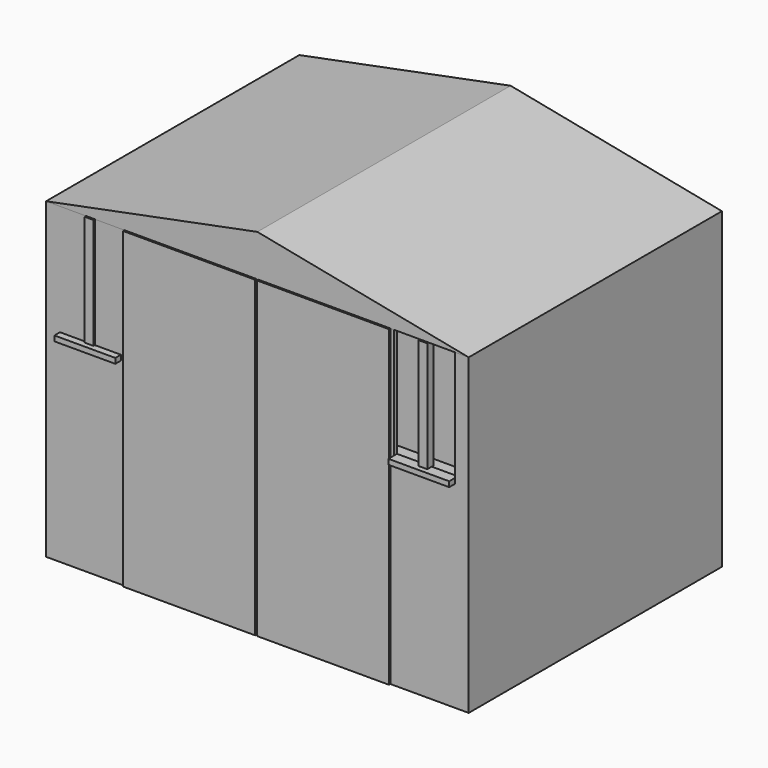
from build123d import *

# Parameters (mm, degrees)
F0_W          = 243
F0_H          = 182
F0_W_2        = 238.6
F0_H_2        = 177.6
F1_DEPTH      = 180
F2_DEPTH      = 2.2
F3_W          = 76
F3_H          = 180
F3_W_2        = 5
F3_H_2        = 63.7124854326
F4_DEPTH      = 1
F4_DEPTH_BACK = 3.3
F3_W_3        = 15
F5_DEPTH      = 25
F6_DEPTH      = 8
F7_DEPTH      = 4
F9_DEPTH      = 182


# Not quite as in the source:
# - a feature names something its author has since deleted; it is built from what else it names


with BuildPart() as f1:
    # F0 (on Top) → F1 (new body)
    with BuildSketch(Plane.XY):
        with Locations((121.5, -91)):
            Rectangle(F0_W, F0_H)
        with Locations((121.5, -91)):
            Rectangle(F0_W_2, F0_H_2, mode=Mode.SUBTRACT)
    extrude(amount=F1_DEPTH)

    # F0 (on Top) → F2 (join)
    with BuildSketch(Plane.XY):
        with Locations((121.5, -91)):
            Rectangle(F0_W_2, F0_H_2)
    extrude(amount=F2_DEPTH)

    # F3 (on face) → F4 (join, two sides)
    with BuildSketch(Plane.XZ.offset(182)) as f4_sk:
        with Locations((83, 90)):
            Rectangle(F3_W, F3_H)
        with Locations((160, 90)):
            Rectangle(F3_W, F3_H)
        with Locations((25.5, 148.1437572837)):
            Rectangle(F3_W_2, F3_H_2)
        with Locations((217.5, 148.1437572837)):
            Rectangle(F3_W_2, F3_H_2)
    extrude(amount=F4_DEPTH)
    extrude(f4_sk.sketch, amount=-F4_DEPTH_BACK)

    # F3 (on face) → F5 (cut)
    with BuildSketch(Plane.XZ.offset(182)):
        Polygon((43, 180), (45, 180), (121, 180), (122, 180), (198, 180), (200, 180), (215, 180), (220, 180), (235, 180), (243, 180), (121.5, 204), (0, 180), (8, 180), (23, 180), (28, 180), align=None)
        with Locations((207.5, 148.1437572837)):
            Rectangle(F3_W_3, F3_H_2)
        with Locations((227.5, 148.1437572837)):
            Rectangle(F3_W_3, F3_H_2)
    extrude(amount=-F5_DEPTH, mode=Mode.SUBTRACT)

    # F3 (on face) → F6 (join)
    with BuildSketch(Plane.XZ.offset(182)):
        Polygon((43, 180), (45, 180), (121, 180), (122, 180), (198, 180), (200, 180), (215, 180), (220, 180), (235, 180), (243, 180), (121.5, 204), (0, 180), (8, 180), (23, 180), (28, 180), align=None)
    extrude(amount=-F6_DEPTH)

    # F3 (on face) → F7 (join)
    with BuildSketch(Plane.XZ.offset(182)):
        Polygon((215, 116.2875145674), (200, 116.2875145674), (200, 113.2875145674), (235, 113.2875145674), (235, 116.2875145674), (220, 116.2875145674), align=None)
        Polygon((43, 113.2875145674), (43, 116.2875145674), (28, 116.2875145674), (23, 116.2875145674), (8, 116.2875145674), (8, 113.2875145674), align=None)
    extrude(amount=F7_DEPTH)


with BuildPart() as f9:
    # F8 (on face) → F9 (new body)
    with BuildSketch(Plane(origin=(0, 0, 0), x_dir=(-1, 0, 0), z_dir=(0, 1, 0))):
        Polygon((-121.5, 204), (-243, 180), (0, 180), align=None)
    extrude(amount=-F9_DEPTH)


solid = Compound([f1.part, f9.part])
